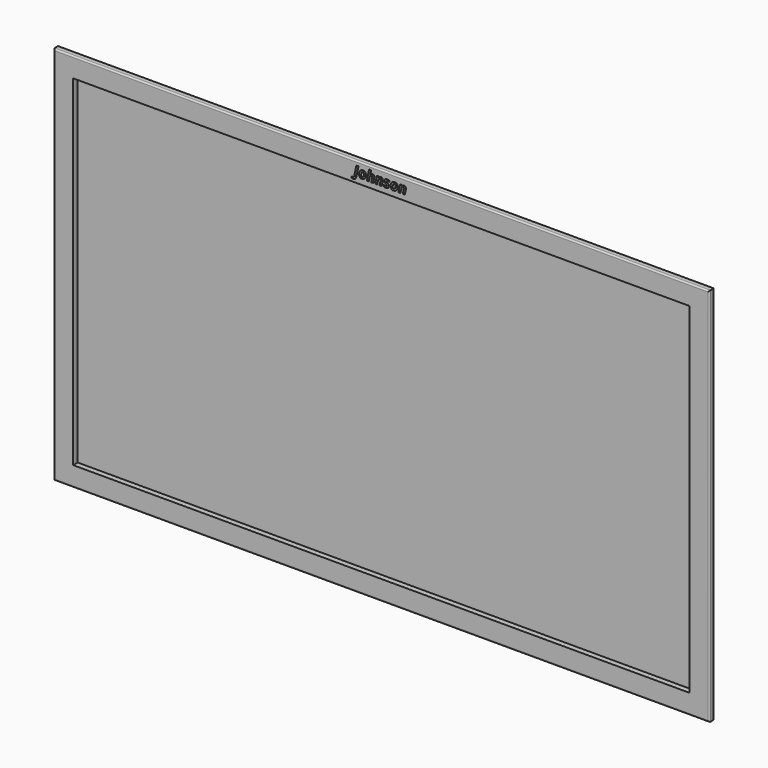
from build123d import *

# Parameters (mm, degrees)
F0_W         = 2781.3
F0_H         = 1536.7
F1_DEPTH     = 0.254
F2_W         = 2679.7
F2_H         = 38.1
F2_W_2       = 88.9
F2_H_2       = 1435.1
F3_DEPTH     = 25.4
F4_W         = 2959.1
F4_H         = 1714.5
F4_W_2       = 2781.3
F4_H_2       = 1536.7
F5_DEPTH     = 25.4
F6_R         = 6.35
F7_TEXT_SIZE = 62.956419771
F8_DEPTH     = 51.055


# Not quite as in the source:
# - Text() gives the source's letters only with a copy of the font that has no kerning and outlines rounded to 1/6400 em; it was checked with that copy


with BuildPart() as f1:
    # F0 (on Front) → F1 (new body)
    with BuildSketch(Plane.XZ):
        Rectangle(F0_W, F0_H)
    extrude(amount=F1_DEPTH)

    # F2 (on face) → F3 (join)
    with BuildSketch(Plane(origin=(0, 0, 0), x_dir=(-1, 0, 0), z_dir=(0, 1, 0))):
        Polygon((-1339.85, 806.45), (-1428.75, 806.45), (-1428.75, -806.45), (-1339.85, -806.45), (-1339.85, -768.35), (-1390.65, -768.35), (-1390.65, 768.35), (-1339.85, 768.35), align=None)
        Polygon((-1339.85, 717.55), (-1339.85, 768.35), (-1390.65, 768.35), (-1390.65, -768.35), (-1339.85, -768.35), (-1339.85, -717.55), align=None)
        Polygon((1339.85, 768.35), (-1339.85, 768.35), (-1339.85, 717.55), (-44.45, 717.55), (44.45, 717.55), (1339.85, 717.55), align=None)
        with Locations((0, 787.4)):
            Rectangle(F2_W, F2_H)
        Polygon((1428.75, 806.45), (1339.85, 806.45), (1339.85, 768.35), (1390.65, 768.35), (1390.65, -768.35), (1339.85, -768.35), (1339.85, -806.45), (1428.75, -806.45), align=None)
        with Locations((0, -787.4)):
            Rectangle(F2_W, F2_H)
        Polygon((1390.65, 768.35), (1339.85, 768.35), (1339.85, 717.55), (1339.85, -717.55), (1339.85, -768.35), (1390.65, -768.35), align=None)
        Polygon((-1339.85, -717.55), (-1339.85, -768.35), (1339.85, -768.35), (1339.85, -717.55), (44.45, -717.55), (-44.45, -717.55), align=None)
        Rectangle(F2_W_2, F2_H_2)
    extrude(amount=F3_DEPTH)


with BuildPart() as f5:
    # F4 (on face) → F5 (new body)
    with BuildSketch(Plane.XZ.offset(0.254)):
        Rectangle(F4_W, F4_H)
        Rectangle(F4_W_2, F4_H_2, mode=Mode.SUBTRACT)
    extrude(amount=F5_DEPTH)

    # F6
    f6_edges = [f5.edges().sort_by_distance(p)[0] for p in [
        (0, -25.654, 857.25),
        (-1479.55, -25.654, 0),
        (0, -25.654, -857.25),
        (1479.55, -25.654, 0),
    ]]
    fillet(f6_edges, radius=F6_R)

    # F7 (on face) → F8 (cut, through all)
    with BuildSketch(Plane.XZ.offset(25.654)):
        with Locations((-124.5799340921, 792.8713777649)):
            Text('Johnson', F7_TEXT_SIZE, font='Open Sans', font_style=FontStyle.BOLDITALIC, text_align=(TextAlign.LEFT, TextAlign.BOTTOM))
    extrude(amount=-F8_DEPTH, mode=Mode.SUBTRACT)


solid = Compound([f1.part, f5.part])
